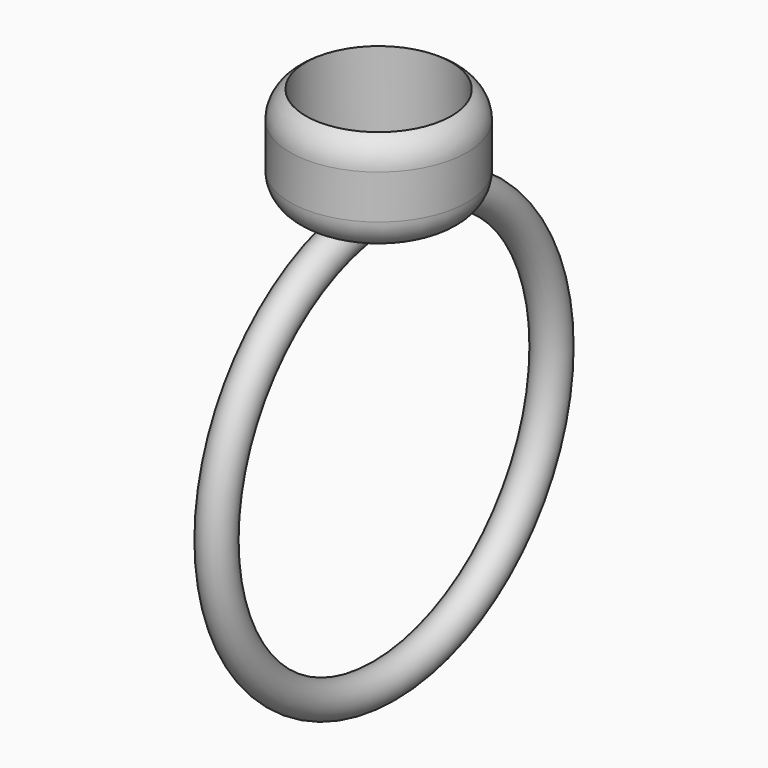
from build123d import *

# Parameters (mm, degrees)
F1_R     = 2.7469010715
F4_R     = 14.0819021009
F5_DEPTH = 16.25
F6_T     = -2.5


# Not quite as in the source:
# - a fillet or chamfer that OpenCascade refuses, or shapes differently, is made with other operations: its cross-section is extruded or revolved along the edge and cut away or added


with BuildPart() as f2:
    # F2: sweep along a path in F0
    with BuildLine(Plane.YZ) as f2_path:
        CenterArc((0, 0), 34.0842518569, 0, 360)
    # F1 (on Top) → F2 (sweep)
    with BuildSketch(Plane.XY):
        with Locations((0, 33.305324614)):
            Circle(F1_R)
    sweep(path=f2_path.line)


with BuildPart() as f5:
    # F4 (on offset) → F5 (new body)
    with BuildSketch(Plane.XY.offset(50)):
        with Locations((0, -1.069550286)):
            Circle(F4_R)
    extrude(amount=-F5_DEPTH)

    # F6
    f6_openings = [f5.faces().sort_by_distance(p)[0] for p in [
        (0, -1.06955, 50),
    ]]
    offset(amount=F6_T, openings=f6_openings)

    # F7: fillet of radius 5 on 2 edges, made by hand

    # F7_s1 → F7_t2 (revolve, cut)
    with BuildSketch(Plane.XZ.offset(1.069550286)):
        with BuildLine():
            ThreePointArc((14.0820521009, 45.6699595845), (13.4121574685, 48.1699970853), (11.5819770987, 50.0001299051))
            Line((11.5819770987, 50.0001299051), (11.6319755986, 50.0867333115))
            ThreePointArc((11.6319755986, 50.0867333115), (12.8319395998, 50.1), (14.0819021009, 50.1))
            Line((14.0819021009, 50.1), (14.1819021009, 50))
            ThreePointArc((14.1819021009, 50), (14.1819021009, 47.8349797922), (14.1820521009, 45.6699595845))
            Line((14.1820521009, 45.6699595845), (14.0820521009, 45.6699595845))
        make_face()
    revolve(axis=Axis((0, -1.069550286, 50), (0, 0, 1)), mode=Mode.SUBTRACT)

    # F7_s3 → F7_t4 (revolve, cut)
    with BuildSketch(Plane.XZ.offset(1.069550286)):
        with BuildLine():
            ThreePointArc((14.0820521009, 38.74985), (12.6175860068, 35.2143160941), (9.0820521009, 33.74985))
            Line((9.0820521009, 33.74985), (9.0820521009, 33.64985))
            ThreePointArc((9.0820521009, 33.64985), (11.5819771009, 33.65), (14.0819021009, 33.65))
            Line((14.0819021009, 33.65), (14.1819021009, 33.75))
            ThreePointArc((14.1819021009, 33.75), (14.1819021009, 36.249925), (14.1820521009, 38.74985))
            Line((14.1820521009, 38.74985), (14.0820521009, 38.74985))
        make_face()
    revolve(axis=Axis((0, -1.069550286, 33.75), (0, 0, 1)), mode=Mode.SUBTRACT)


solid = Compound([f2.part, f5.part])
